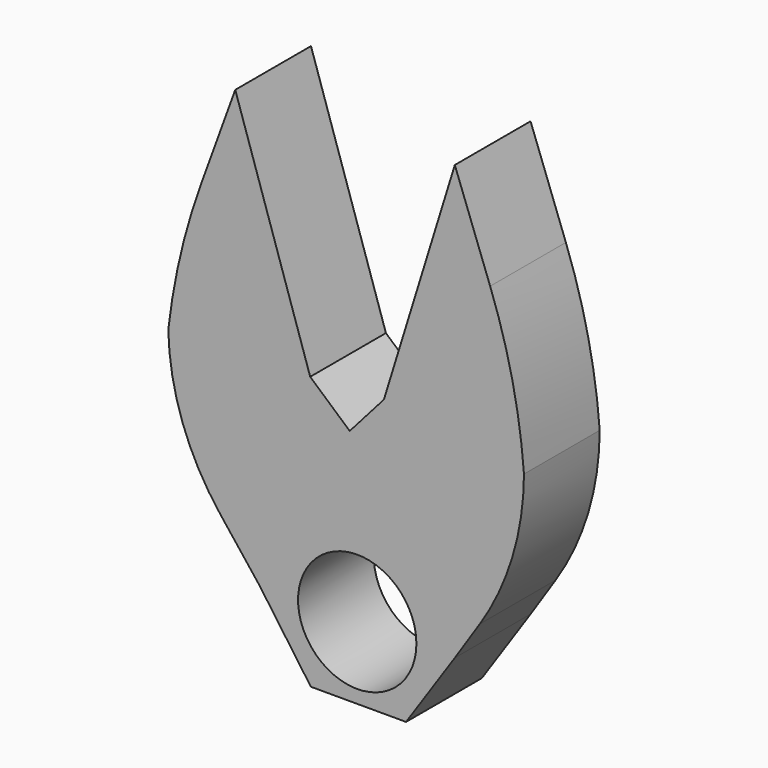
from build123d import *

# Parameters (mm, degrees)
F1_DEPTH    = 203.2
F2_R        = 524.2150172708
F3_R        = 576.4720659651
F4_T1_DEPTH = 1259.1165686585
F5_T1_DEPTH = 1255.3749905901


# Not quite as in the source:
# - a fillet or chamfer that OpenCascade refuses, or shapes differently, is made with other operations: its cross-section is extruded or revolved along the edge and cut away or added


with BuildPart() as f1:
    # F0 (on Front) → F1 (new body)
    with BuildSketch(Plane.XZ):
        with BuildLine():
            ThreePointArc((-110.8744768228, -261.0464180114), (16.1255231772, -134.0464180114), (143.1255231772, -261.0464180114))
            Line((143.1255231772, -261.0464180114), (225.592463352, -261.0464180114))
            Line((225.592463352, -261.0464180114), (373.2602894306, -36.582775414))
            Line((373.2602894306, -36.582775414), (374.6494054794, 268.6479091644))
            Line((374.6494054794, 268.6479091644), (225.592463352, 670.33340462))
            Line((225.592463352, 670.33340462), (73.3804965445, 177.5454695022))
            Line((73.3804965445, 177.5454695022), (0, 94.2992939619))
            Line((0, 94.2992939619), (-84.8674460535, 169.1089208481))
            Line((-84.8674460535, 169.1089208481), (-245.7081394527, 659.1119712874))
            Line((-245.7081394527, 659.1119712874), (-391.4476633072, 258.2389712334))
            Line((-391.4476633072, 258.2389712334), (-385.8949542046, -15.7268568873))
            Line((-385.8949542046, -15.7268568873), (-193.3414169976, -261.0464180114))
            Line((-193.3414169976, -261.0464180114), (-110.8744768228, -261.0464180114))
        make_face()
        with BuildLine():
            Line((225.592463352, -261.0464180114), (143.1255231772, -261.0464180114))
            ThreePointArc((143.1255231772, -261.0464180114), (16.1255231772, -388.0464180114), (-110.8744768228, -261.0464180114))
            Line((-110.8744768228, -261.0464180114), (-193.3414169976, -261.0464180114))
            Line((-193.3414169976, -261.0464180114), (-83.4842249751, -416.1604046822))
            Line((-83.4842249751, -416.1604046822), (120.9037303925, -416.1604046822))
            Line((120.9037303925, -416.1604046822), (225.592463352, -261.0464180114))
        make_face()
    extrude(amount=F1_DEPTH)

    # F2
    f2_edges = [f1.edges().sort_by_distance(p)[0] for p in [
        (-385.894954, -101.6, -15.726857),
    ]]
    fillet(f2_edges, radius=F2_R)

    # F3
    f3_edges = [f1.edges().sort_by_distance(p)[0] for p in [
        (373.260289, -101.6, -36.582775),
    ]]
    fillet(f3_edges, radius=F3_R)

    # F4: fillet of radius 1309.0101889576 on 1 edges, made by hand

    # F4_s2 → F4_t1 (cut)
    with BuildSketch(Plane.XZ.offset(-527.9582843292)):
        with BuildLine():
            ThreePointArc((-389.4458686955, 159.4721695887), (-363.0670592886, 310.1454864879), (-319.291432217, 456.7128242054))
            Line((-319.291432217, 456.7128242054), (-391.4476633072, 258.2389712334))
            Line((-391.4476633072, 258.2389712334), (-389.4458686955, 159.4721695887))
        make_face()
    extrude(amount=F4_T1_DEPTH, mode=Mode.SUBTRACT)

    # F5: fillet of radius 1218.6389974417 on 1 edges, made by hand

    # F5_s2 → F5_t1 (cut)
    with BuildSketch(Plane.XZ.offset(-526.087495295)):
        with BuildLine():
            ThreePointArc((301.4394303457, 465.9375134872), (349.3234640421, 302.8101982001), (374.039377549, 134.6063775081))
            Line((374.039377549, 134.6063775081), (374.6494054794, 268.6479091644))
            Line((374.6494054794, 268.6479091644), (301.4394303457, 465.9375134872))
        make_face()
    extrude(amount=F5_T1_DEPTH, mode=Mode.SUBTRACT)


solid = f1.part
